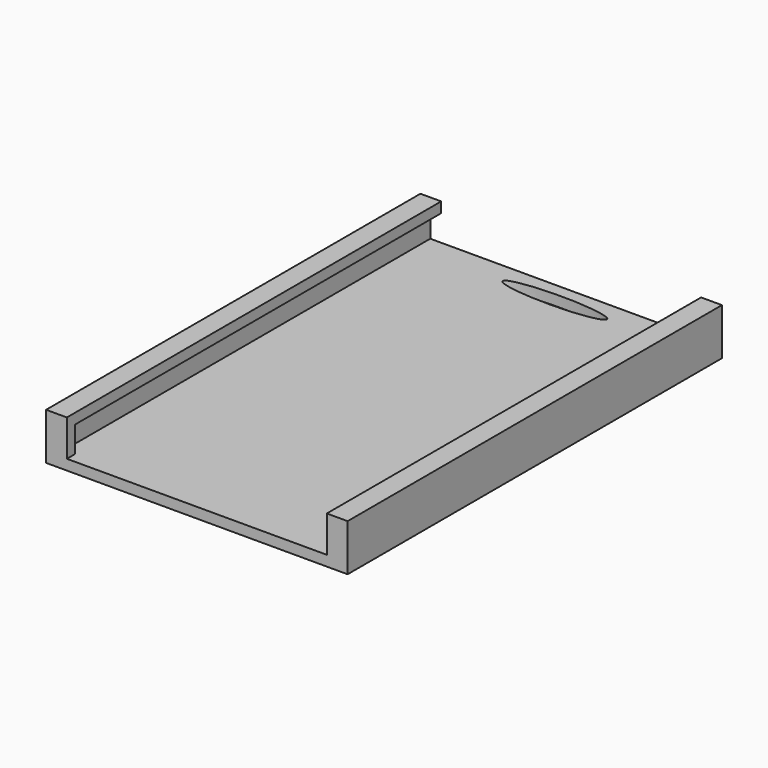
from build123d import *

# Parameters (mm, degrees)
F0_W     = 58
F0_H     = 90
F1_DEPTH = 9
F2_W     = 50
F2_H     = 90
F3_DEPTH = 7
F4_W     = 54.2
F4_H     = 5
F5_DEPTH = 88
F7_DEPTH = 25


# Not quite as in the source:
# - a feature names something its author has since deleted; it is built from what else it names


with BuildPart() as f1:
    # F0 (on Top) → F1 (new body)
    with BuildSketch(Plane.XY):
        Rectangle(F0_W, F0_H)
    extrude(amount=F1_DEPTH)

    # F2 (on face) → F3 (cut)
    with BuildSketch(Plane.XY.offset(9)):
        Rectangle(F2_W, F2_H)
    extrude(amount=-F3_DEPTH, mode=Mode.SUBTRACT)

    # F4 (on face) → F5 (cut)
    with BuildSketch(Plane(origin=(0, 45, 0), x_dir=(-1, 0, 0), z_dir=(0, 1, 0))):
        with Locations((0, 4.5)):
            Rectangle(F4_W, F4_H)
    extrude(amount=-F5_DEPTH, mode=Mode.SUBTRACT)

    # F6 (on face) → F7 (cut)
    with BuildSketch(Plane.XY.offset(2)):
        with BuildLine():
            add(Edge.make_bspline(
                [(10.0087067112, 41.0774275661), (10.0087067112, 43.8166453426), (-5.0043533556, 42.4470364543), (-20.0174134225, 41.0774275661), (-5.0043533556, 39.7078186778), (10.0087067112, 38.3382097895), (10.0087067112, 41.0774275661)],
                knots=[0, 0, 0, 2.0943951024, 2.0943951024, 4.1887902048, 4.1887902048, 6.2831853072, 6.2831853072, 6.2831853072], degree=2, weights=[1, 0.5, 1, 0.5, 1, 0.5, 1]))
        make_face()
    extrude(amount=-F7_DEPTH, mode=Mode.SUBTRACT)


solid = f1.part
